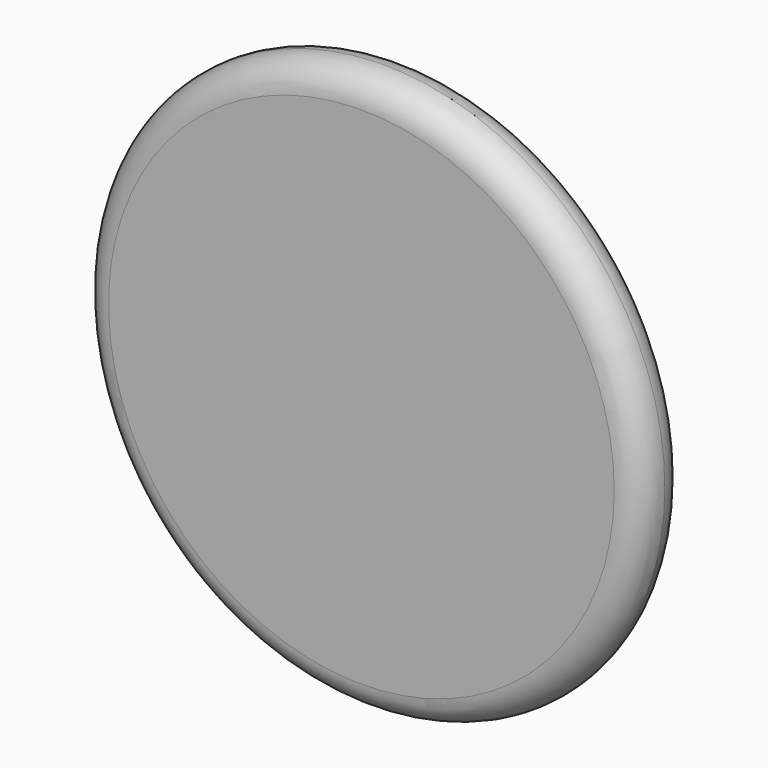
from build123d import *

# Parameters (mm, degrees)
F0_R     = 50
F1_DEPTH = 10
F2_R     = 4.99999


# Not quite as in the source:
# - a fillet or chamfer is up to 0.001 mm smaller than in the source, because OpenCascade refuses the exact size


with BuildPart() as f1:
    # F0 (on Front) → F1 (new body)
    with BuildSketch(Plane.XZ):
        Circle(F0_R)
    extrude(amount=F1_DEPTH)

    # F2 (radius 5 in the source; OpenCascade refuses exactly that, so slightly less here)
    f2_edges = [f1.edges().sort_by_distance(p)[0] for p in [
        (-50, -10, 0),
        (-50, 0, 0),
    ]]
    fillet(f2_edges, radius=F2_R)


solid = f1.part
